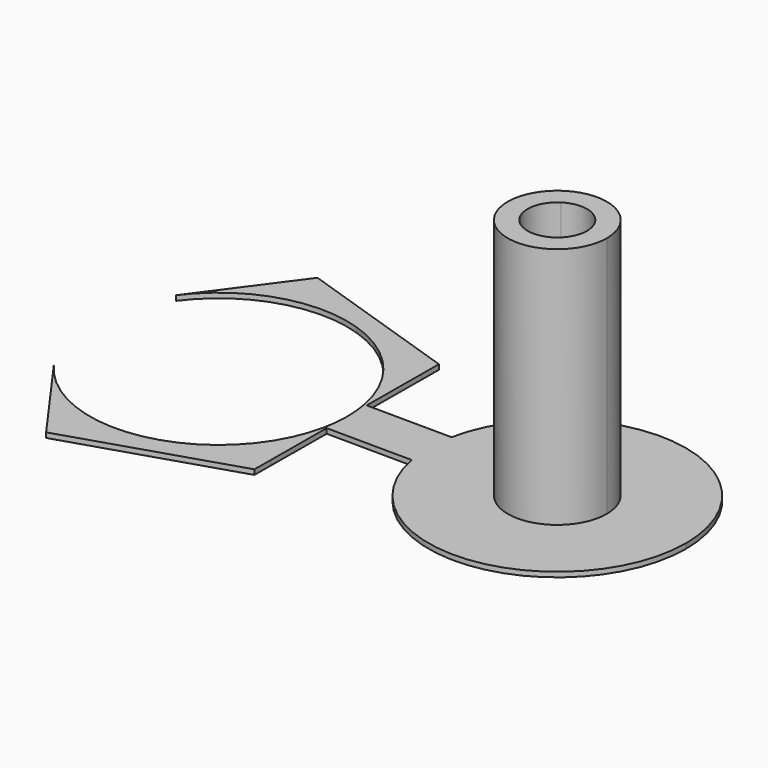
from build123d import *

# Parameters (mm, degrees)
F1_DEPTH = 0.5
F2_DEPTH = 25
F3_R     = 2.9
F4_DEPTH = 0.501
F6_DEPTH = 0.5


# Not quite as in the source:
# - a feature names something its author has since deleted; it is built from what else it names


with BuildPart() as f1:
    # F0 (on Top) → F1 (new body)
    with BuildSketch(Plane.XY):
        with BuildLine():
            Line((4.0961373656, 12.3378141776), (-4.8678095704, 15.3138321001))
            Line((-4.8678095704, 15.3138321001), (-10.4681826882, 7.7082521499))
            ThreePointArc((-10.4681826882, 7.7082521499), (-3.9381406197, 12.3891504333), (4.0961373656, 12.3378141776))
        make_face()
    extrude(amount=F1_DEPTH)



with BuildPart() as f1b:
    # F0 (on Top) → F1, piece 2 (new body)
    with BuildSketch(Plane.XY):
        with BuildLine():
            Line((13.0600839256, 9.36179638), (4.0961373656, 12.3378141776))
            ThreePointArc((4.0961373656, 12.3378141776), (9.7852826172, 8.5585188031), (12.7733744664, 2.41679638))
            Line((12.7733744664, 2.41679638), (13.01569776, 2.4152179267))
            Line((13.01569776, 2.4152179267), (13.0600839256, 9.36179638))
        make_face()
        with BuildLine():
            Line((13.01569776, 2.4152179267), (12.7733744664, 2.41679638))
            ThreePointArc((12.7733744664, 2.41679638), (12.9432196161, 1.2136992909), (13, 0))
            ThreePointArc((13, 0), (12.9999336569, -0.0415321088), (12.9997346283, -0.0830637936))
            Line((12.9997346283, -0.0830637936), (13.01569776, 2.4152179267))
        make_face()
        with BuildLine():
            Line((21.6332001204, 2.3590849609), (13.01569776, 2.4152179267))
            Line((13.01569776, 2.4152179267), (12.9997346283, -0.0830637936))
            Line((12.9997346283, -0.0830637936), (12.9837495259, -2.5847840032))
            Line((12.9837495259, -2.5847840032), (21.6006561013, -2.640828477))
            ThreePointArc((21.6006561013, -2.640828477), (21.374282177, -0.1392923959), (21.6332001204, 2.3590849609))
        make_face()
        with BuildLine():
            ThreePointArc((12.7407636764, -2.58320362), (9.6739656437, -8.6841458259), (3.9381407553, -12.3891503902))
            Line((3.9381407553, -12.3891503902), (12.9393853324, -9.5279237416))
            Line((12.9393853324, -9.5279237416), (12.9837495259, -2.5847840032))
            Line((12.9837495259, -2.5847840032), (12.7407636764, -2.58320362))
        make_face()
        with BuildLine():
            Line((12.9837495259, -2.5847840032), (12.9997346283, -0.0830637936))
            ThreePointArc((12.9997346283, -0.0830637936), (12.9308154434, -1.3394073199), (12.7407636764, -2.58320362))
            Line((12.7407636764, -2.58320362), (12.9837495259, -2.5847840032))
        make_face()
        with BuildLine():
            ThreePointArc((47.3740068068, -0.2239065181), (35.6719885241, 12.7111328503), (21.6332001204, 2.3590849609))
            Line((21.6332001204, 2.3590849609), (30.0602249194, 2.304192734))
            ThreePointArc((30.0602249194, 2.304192734), (35.6837950651, 4.6014903276), (39.3740068068, -0.2239065181))
            ThreePointArc((39.3740068068, -0.2239065181), (35.6523599398, -5.0577262569), (30.0276814999, -2.6956379611))
            Line((30.0276814999, -2.6956379611), (21.6006561013, -2.640828477))
            ThreePointArc((21.6006561013, -2.640828477), (35.5877697221, -13.1671201679), (47.3740068068, -0.2239065181))
        make_face()
        with BuildLine():
            Line((30.0602249194, 2.304192734), (21.6332001204, 2.3590849609))
            ThreePointArc((21.6332001204, 2.3590849609), (21.374282177, -0.1392923959), (21.6006561013, -2.640828477))
            Line((21.6006561013, -2.640828477), (30.0276814999, -2.6956379611))
            ThreePointArc((30.0276814999, -2.6956379611), (29.374112718, -0.1913626859), (30.0602249194, 2.304192734))
        make_face()
        with BuildLine():
            Line((32.7319335315, 2.286789672), (30.0602249194, 2.304192734))
            ThreePointArc((30.0602249194, 2.304192734), (29.374112718, -0.1913626859), (30.0276814999, -2.6956379611))
            Line((30.0276814999, -2.6956379611), (32.6993904313, -2.7130147911))
            ThreePointArc((32.6993904313, -2.7130147911), (31.3740703529, -0.2043803079), (32.7319335315, 2.286789672))
        make_face()
        with BuildLine():
            ThreePointArc((37.3740068068, -0.2239065181), (35.80120339, 2.4148640125), (32.7319335315, 2.286789672))
            Line((32.7319335315, 2.286789672), (34.3740068068, 2.2760934819))
            Line((34.3740068068, 2.2760934819), (34.3740068068, -2.7239065181))
            Line((34.3740068068, -2.7239065181), (32.6993904313, -2.7130147911))
            ThreePointArc((32.6993904313, -2.7130147911), (35.7839980964, -2.8719104009), (37.3740068068, -0.2239065181))
        make_face()
        with BuildLine():
            Line((34.3740068068, 2.2760934819), (32.7319335315, 2.286789672))
            ThreePointArc((32.7319335315, 2.286789672), (31.3740703529, -0.2043803079), (32.6993904313, -2.7130147911))
            Line((32.6993904313, -2.7130147911), (34.3740068068, -2.7239065181))
            Line((34.3740068068, -2.7239065181), (34.3740068068, 2.2760934819))
        make_face()
    extrude(amount=F1_DEPTH)

    # F0 (on Top) → F2 (join)
    with BuildSketch(Plane.XY):
        with BuildLine():
            ThreePointArc((39.3740068068, -0.2239065181), (35.6837950651, 4.6014903276), (30.0602249194, 2.304192734))
            Line((30.0602249194, 2.304192734), (32.7319335315, 2.286789672))
            ThreePointArc((32.7319335315, 2.286789672), (35.80120339, 2.4148640125), (37.3740068068, -0.2239065181))
            ThreePointArc((37.3740068068, -0.2239065181), (35.7839980964, -2.8719104009), (32.6993904313, -2.7130147911))
            Line((32.6993904313, -2.7130147911), (30.0276814999, -2.6956379611))
            ThreePointArc((30.0276814999, -2.6956379611), (35.6523599398, -5.0577262569), (39.3740068068, -0.2239065181))
        make_face()
        with BuildLine():
            Line((32.7319335315, 2.286789672), (30.0602249194, 2.304192734))
            ThreePointArc((30.0602249194, 2.304192734), (29.374112718, -0.1913626859), (30.0276814999, -2.6956379611))
            Line((30.0276814999, -2.6956379611), (32.6993904313, -2.7130147911))
            ThreePointArc((32.6993904313, -2.7130147911), (31.3740703529, -0.2043803079), (32.7319335315, 2.286789672))
        make_face()
    extrude(amount=F2_DEPTH)

    # F3 (on face) → F4 (cut, through all)
    with BuildSketch(Plane.XY.offset(0.5)):
        with Locations((34.3740068068, -0.2239065181)):
            Circle(F3_R)
    extrude(amount=-F4_DEPTH, mode=Mode.SUBTRACT)


with BuildPart() as f1c:
    # F0 (on Top) → F1, piece 3 (new body)
    with BuildSketch(Plane.XY):
        with BuildLine():
            ThreePointArc((3.9381407553, -12.3891503902), (-4.096137147, -12.3378142502), (-10.5658298597, -7.5738523471))
            Line((-10.5658298597, -7.5738523471), (-5.0631039967, -15.2503770945))
            Line((-5.0631039967, -15.2503770945), (3.9381407553, -12.3891503902))
        make_face()
    extrude(amount=F1_DEPTH)


with BuildPart() as f1_1:
    add(f1.part)

    add(f1b.part)  # F6 merges F1b

    add(f1c.part)  # F6 merges F1c
    # F5 (on face) → F6 (join, through all)
    with BuildSketch(Plane.XY):
        Polygon((-4.8678095704, 15.3138321001), (4.0961371776, 12.3378142401), (13.0600839256, 9.36179638), (13.0735205907, 11.4646779011), (-3.6208963346, 17.0072011144), align=None)
        Polygon((-5.0631039967, -15.2503770945), (-3.8421437919, -16.9585881221), (12.9230595755, -11.6340152664), (12.9393853324, -9.5279237416), (3.9381406679, -12.389150418), align=None)
    extrude(amount=F6_DEPTH)


solid = f1_1.part
